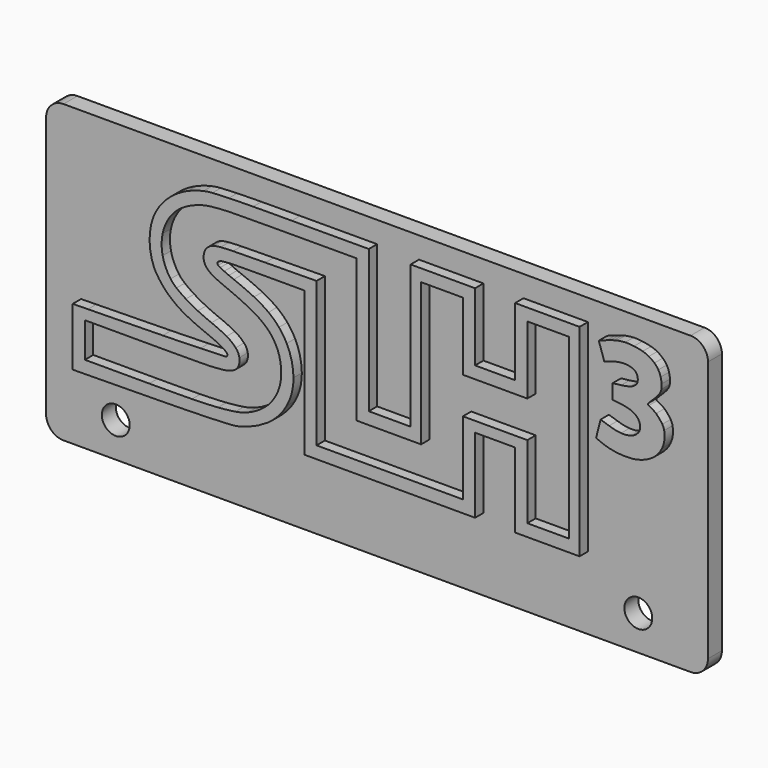
from build123d import *

# Parameters (mm, degrees)
F1_DEPTH = 6
F2_W     = 380
F2_H     = 170
F2_R     = 8
F3_DEPTH = 10
F4_R     = 10


# Not quite as in the source:
# - ends of sketch curves that miss each other by under 0.0002 mm in the source are joined


with BuildPart() as f1:
    # F0 (on Front) → F1 (new body)
    with BuildSketch(Plane.XZ):
        with BuildLine():
            ThreePointArc((152.341228018, 58.1349171313), (149.8269064082, 58.3597525344), (147.3038345575, 58.4402047098))
            ThreePointArc((147.3038345575, 58.4402047098), (144.8923426463, 58.2191881424), (142.5041551762, 57.818311393))
            ThreePointArc((142.5041551762, 57.818311393), (141.6286371814, 57.5874283564), (140.7541334629, 57.352732867))
            ThreePointArc((140.7541334629, 57.352732867), (139.7941303297, 57.0530705945), (138.8354301453, 56.749265641))
            ThreePointArc((138.8354301453, 56.749265641), (137.8311964898, 56.4206441356), (136.8284840268, 56.0874099159))
            ThreePointArc((136.8284840268, 56.0874099159), (134.4494339346, 55.2578316154), (132.1058124304, 54.3328896165))
            Line((132.1058124304, 54.3328896165), (135.2964043617, 44.7889044881))
            ThreePointArc((135.2964043617, 44.7889044881), (138.9218950311, 46.1431942866), (142.6777168508, 47.0770496879))
            ThreePointArc((142.6777168508, 47.0770496879), (145.3037154455, 47.4599296937), (147.9574100047, 47.4791820766))
            ThreePointArc((147.9574100047, 47.4791820766), (150.0024260919, 47.1622128392), (151.9545679078, 46.4754067993))
            ThreePointArc((151.9545679078, 46.4754067993), (153.2497169486, 45.5413952884), (154.0946016381, 44.1864198624))
            ThreePointArc((154.0946016381, 44.1864198624), (154.4618796803, 42.6793722604), (154.4471411344, 41.1282859819))
            ThreePointArc((154.4471411344, 41.1282859819), (154.0274505966, 39.8196352665), (153.1810760747, 38.7368809167))
            ThreePointArc((153.1810760747, 38.7368809167), (151.7322273647, 37.7109786626), (150.0881481192, 37.0411715732))
            ThreePointArc((150.0881481192, 37.0411715732), (147.5640252841, 36.4404230958), (145.0010969923, 36.0360800651))
            Line((145.0010969923, 36.0360800651), (140.077451, 35.452947))
            Line((140.077451, 35.452947), (140.077451, 31.231529))
            Line((140.077451, 31.231529), (140.077451, 27.010111))
            Line((140.077451, 27.010111), (145.313272, 26.390005))
            ThreePointArc((145.313272, 26.390005), (147.4995114305, 26.0344391507), (149.6467600868, 25.4909382897))
            ThreePointArc((149.6467600868, 25.4909382897), (151.3253195044, 24.8379266625), (152.8788301944, 23.9265592779))
            ThreePointArc((152.8788301944, 23.9265592779), (154.0260482227, 22.9373393661), (154.9508350367, 21.7375750228))
            ThreePointArc((154.9508350367, 21.7375750228), (155.5731072533, 20.4211762125), (155.8821842516, 18.9982919249))
            ThreePointArc((155.8821842516, 18.9982919249), (155.6792998869, 16.9086609443), (154.6903602154, 15.0567108232))
            ThreePointArc((154.6903602154, 15.0567108232), (152.9583603485, 13.4737955374), (150.8501020813, 12.4438967473))
            ThreePointArc((150.8501020813, 12.4438967473), (147.9002641766, 11.809008744), (144.8831400017, 11.7691580196))
            ThreePointArc((144.8831400017, 11.7691580196), (141.4066010267, 12.2925822347), (138.0238769802, 13.2504309438))
            Line((138.0238769802, 13.2504309438), (133.1239811244, 14.812147956))
            Line((133.1239811244, 14.812147956), (130.5830776691, 4.6951826662))
            ThreePointArc((130.5830776691, 4.6951826662), (134.3545111151, 3.0830213335), (138.2702710743, 1.8625303084))
            ThreePointArc((138.2702710743, 1.8625303084), (144.6475148349, 0.8652287383), (151.1020819971, 0.9143360329))
            ThreePointArc((151.1020819971, 0.9143360329), (156.7168065495, 2.0783580357), (161.91616203, 4.4963699511))
            ThreePointArc((161.91616203, 4.4963699511), (165.7064525048, 7.6555621469), (168.4426272472, 11.7616728825))
            ThreePointArc((168.4426272472, 11.7616728825), (169.7953031287, 16.3544948874), (169.6605109651, 21.1404719934))
            ThreePointArc((169.6605109651, 21.1404719934), (169.2435398041, 22.6044121534), (168.5656666596, 23.9673037896))
            ThreePointArc((168.5656666596, 23.9673037896), (166.9064128382, 26.1972938101), (165.0162637234, 28.2352622598))
            ThreePointArc((165.0162637234, 28.2352622598), (162.9669138924, 29.6544963373), (160.7904410002, 30.8698258589))
            ThreePointArc((160.7904410002, 30.8698258589), (160.3825279534, 31.451864804), (160.663634351, 32.1046600097))
            ThreePointArc((160.663634351, 32.1046600097), (162.3630635173, 33.8079757087), (164.0774507347, 35.4962352653))
            ThreePointArc((164.0774507347, 35.4962352653), (165.1707236148, 36.6322034695), (166.2196933125, 37.809204732))
            ThreePointArc((166.2196933125, 37.809204732), (166.8414404287, 38.6357965203), (167.3527699769, 39.5348880112))
            ThreePointArc((167.3527699769, 39.5348880112), (167.8080801222, 40.4998853929), (168.087775057, 41.5295931274))
            ThreePointArc((168.087775057, 41.5295931274), (168.1977643706, 42.8800995541), (168.1963354349, 44.2350767553))
            ThreePointArc((168.1963354349, 44.2350767553), (167.9958020572, 45.8752345594), (167.6282000052, 47.4861970012))
            ThreePointArc((167.6282000052, 47.4861970012), (167.0891813187, 49.1526573167), (166.3039485131, 50.7182373082))
            ThreePointArc((166.3039485131, 50.7182373082), (165.2790917625, 52.1671747641), (164.0500026364, 53.4474447096))
            ThreePointArc((164.0500026364, 53.4474447096), (162.513830675, 54.6803953844), (160.8520869325, 55.7380338798))
            ThreePointArc((160.8520869325, 55.7380338798), (159.1271747087, 56.5645242409), (157.3094311562, 57.1596856085))
            ThreePointArc((157.3094311562, 57.1596856085), (154.8393231071, 57.7185897611), (152.341228018, 58.1349171313))
        make_face()
    extrude(amount=F1_DEPTH)


with BuildPart() as f1b:
    # F0 (on Front) → F1, piece 2 (new body)
    with BuildSketch(Plane.XZ):
        with BuildLine():
            ThreePointArc((-89.7158710092, 56.8834551585), (-92.2735942046, 56.6347400971), (-94.8042470377, 56.1879701736))
            ThreePointArc((-94.8042470377, 56.1879701736), (-99.3736938541, 54.9568862269), (-103.7987699924, 53.2793543903))
            ThreePointArc((-103.7987699924, 53.2793543903), (-107.8572904997, 51.2349120693), (-111.665558992, 48.7553104477))
            ThreePointArc((-111.665558992, 48.7553104477), (-115.0425226555, 45.9681171918), (-118.0767520571, 42.8112545453))
            ThreePointArc((-118.0767520571, 42.8112545453), (-121.12070834, 38.6532182392), (-123.4993151686, 34.0818764963))
            ThreePointArc((-123.4993151686, 34.0818764963), (-125.7717067995, 20.9710825795), (-123.0967220919, 7.9364695178))
            ThreePointArc((-123.0967220919, 7.9364695178), (-120.9885218169, 4.3857057485), (-118.5278910102, 1.0694235263))
            ThreePointArc((-118.5278910102, 1.0694235263), (-115.7462308189, -1.9692311529), (-112.6660909179, -4.7048835193))
            ThreePointArc((-112.6660909179, -4.7048835193), (-108.9951941367, -7.3754936141), (-105.0961528177, -9.7003846329))
            ThreePointArc((-105.0961528177, -9.7003846329), (-100.2941341921, -12.1054997132), (-95.3662908353, -14.2409905891))
            ThreePointArc((-95.3662908353, -14.2409905891), (-91.8421068748, -15.6870234447), (-88.3419598235, -17.1903045981))
            ThreePointArc((-88.3419598235, -17.1903045981), (-86.1529724976, -18.2297863885), (-84.0291443228, -19.3966375486))
            ThreePointArc((-84.0291443228, -19.3966375486), (-82.7599951917, -20.2264826141), (-81.5746631598, -21.172194182))
            ThreePointArc((-81.5746631598, -21.172194182), (-81.1710412365, -21.8195919106), (-81.1923597658, -22.5822060778))
            ThreePointArc((-81.1923597658, -22.5822060778), (-81.6047236673, -23.1553562233), (-82.2701210101, -23.3915577353))
            ThreePointArc((-82.2701210101, -23.3915577353), (-89.4196222871, -23.6529407729), (-96.5698990129, -23.8921735944))
            ThreePointArc((-96.5698990129, -23.8921735944), (-107.3762638319, -24.1981884626), (-118.1845449963, -24.426714213))
            ThreePointArc((-118.1845449963, -24.426714213), (-139.6783524604, -24.7922369482), (-161.1725489962, -25.1341162467))
            Line((-161.1725489962, -25.1341162467), (-169.922549, -25.268471))
            Line((-169.922549, -25.268471), (-169.922549, -41.902849))
            Line((-169.922549, -41.902849), (-169.922549, -58.537228))
            Line((-169.922549, -58.537228), (-125.172549, -58.013692))
            ThreePointArc((-125.172549, -58.013692), (-115.0424725161, -57.8782248746), (-104.9129060058, -57.7088636826))
            ThreePointArc((-104.9129060058, -57.7088636826), (-97.5129944762, -57.5418252197), (-90.114737023, -57.3129603439))
            ThreePointArc((-90.114737023, -57.3129603439), (-84.6913364364, -57.1009616803), (-79.2697880179, -56.8459516498))
            ThreePointArc((-79.2697880179, -56.8459516498), (-77.083403988, -56.6404610548), (-74.9225491136, -56.2490434966))
            ThreePointArc((-74.9225491136, -56.2490434966), (-66.2429199717, -53.4275060959), (-58.229199749, -49.0597463737))
            ThreePointArc((-58.229199749, -49.0597463737), (-51.8949561555, -43.6034600395), (-47.0349944418, -36.8009257582))
            ThreePointArc((-47.0349944418, -36.8009257582), (-44.1187465301, -29.3501508182), (-43.1776257233, -21.4045329973))
            ThreePointArc((-43.1776257233, -21.4045329973), (-44.2002643647, -13.1406454463), (-47.0554066795, -5.3185108399))
            ThreePointArc((-47.0554066795, -5.3185108399), (-49.0771830946, -1.8182961093), (-51.5059305748, 1.4128443618))
            ThreePointArc((-51.5059305748, 1.4128443618), (-54.3478662536, 4.3900005354), (-57.5111356244, 7.0232085076))
            ThreePointArc((-57.5111356244, 7.0232085076), (-61.5514455995, 9.7367639846), (-65.8219646825, 12.0713206495))
            ThreePointArc((-65.8219646825, 12.0713206495), (-71.5688253864, 14.7325295165), (-77.4225488118, 17.1496274843))
            ThreePointArc((-77.4225488118, 17.1496274843), (-78.8401462889, 17.7131254267), (-80.2487799398, 18.2986711417))
            ThreePointArc((-80.2487799398, 18.2986711417), (-81.6057167765, 18.888922599), (-82.9523677552, 19.5022785255))
            ThreePointArc((-82.9523677552, 19.5022785255), (-84.0942604495, 20.0454792956), (-85.2272229395, 20.6070681197))
            ThreePointArc((-85.2272229395, 20.6070681197), (-85.8377507575, 20.9485781165), (-86.4176780147, 21.3398039801))
            ThreePointArc((-86.4176780147, 21.3398039801), (-86.853730235, 22.0915551847), (-86.6016505259, 22.9232565972))
            ThreePointArc((-86.6016505259, 22.9232565972), (-85.6588933579, 23.6905603449), (-84.5036700444, 24.0687213317))
            ThreePointArc((-84.5036700444, 24.0687213317), (-80.9344247322, 24.4386370453), (-77.3495189905, 24.5961183335))
            ThreePointArc((-77.3495189905, 24.5961183335), (-69.2612379194, 24.6836352737), (-61.1725489995, 24.7162152783))
            Line((-61.1725489995, 24.7162152783), (-36.922549, 24.731529))
            Line((-36.922549, 24.731529), (-36.922549, -16.768471))
            Line((-36.922549, -16.768471), (-36.922549, -58.268471))
            Line((-36.922549, -58.268471), (12.077451, -58.268471))
            Line((12.077451, -58.268471), (61.077451, -58.268471))
            Line((61.077451, -58.268471), (61.077451, -36.768471))
            Line((61.077451, -36.768471), (61.077451, -15.268471))
            Line((61.077451, -15.268471), (72.577451, -15.268471))
            Line((72.577451, -15.268471), (84.077451, -15.268471))
            Line((84.077451, -15.268471), (84.077451, -36.768471))
            Line((84.077451, -36.768471), (84.077451, -58.268471))
            Line((84.077451, -58.268471), (102.577451, -58.268471))
            Line((102.577451, -58.268471), (121.077451, -58.268471))
            Line((121.077451, -58.268471), (121.077451, -0.268471))
            Line((121.077451, -0.268471), (121.077451, 57.731529))
            Line((121.077451, 57.731529), (102.577451, 57.731529))
            Line((102.577451, 57.731529), (84.077451, 57.731529))
            Line((84.077451, 57.731529), (84.077451, 38.231529))
            Line((84.077451, 38.231529), (84.077451, 18.731529))
            Line((84.077451, 18.731529), (72.577451, 18.731529))
            Line((72.577451, 18.731529), (61.077451, 18.731529))
            Line((61.077451, 18.731529), (61.077451, 38.231529))
            Line((61.077451, 38.231529), (61.077451, 57.731529))
            Line((61.077451, 57.731529), (42.577451, 57.731529))
            Line((42.577451, 57.731529), (24.077451, 57.731529))
            Line((24.077451, 57.731529), (24.077451, 16.731529))
            Line((24.077451, 16.731529), (24.077451, -24.268471))
            Line((24.077451, -24.268471), (12.077451, -24.268471))
            Line((12.077451, -24.268471), (0.077451, -24.268471))
            Line((0.077451, -24.268471), (0.077451, 16.731529))
            Line((0.077451, 16.731529), (0.077451, 57.731529))
            Line((0.077451, 57.731529), (-44.172549, 57.652029))
            ThreePointArc((-44.172549, 57.652029), (-55.2418806461, 57.6161162906), (-66.3110620044, 57.5481685759))
            ThreePointArc((-66.3110620044, 57.5481685759), (-73.3088995976, 57.4577720999), (-80.3053760072, 57.2927862479))
            ThreePointArc((-80.3053760072, 57.2927862479), (-85.0121136593, 57.1223791714), (-89.7158710092, 56.8834551585))
        make_face()
        with BuildLine():
            Line((-6.922549, 50.731529), (-6.922549, 9.731529))
            Line((-6.922549, 9.731529), (-6.922549, -31.268471))
            Line((-6.922549, -31.268471), (11.577451, -31.268471))
            Line((11.577451, -31.268471), (30.077451, -31.268471))
            Line((30.077451, -31.268471), (30.077451, 9.731529))
            Line((30.077451, 9.731529), (30.077451, 50.731529))
            Line((30.077451, 50.731529), (42.077451, 50.731529))
            Line((42.077451, 50.731529), (54.077451, 50.731529))
            Line((54.077451, 50.731529), (54.077451, 31.231529))
            Line((54.077451, 31.231529), (54.077451, 11.731529))
            Line((54.077451, 11.731529), (72.577451, 11.731529))
            Line((72.577451, 11.731529), (91.077451, 11.731529))
            Line((91.077451, 11.731529), (91.077451, 31.231529))
            Line((91.077451, 31.231529), (91.077451, 50.731529))
            Line((91.077451, 50.731529), (103.077451, 50.731529))
            Line((103.077451, 50.731529), (115.077451, 50.731529))
            Line((115.077451, 50.731529), (115.077451, -0.268471))
            Line((115.077451, -0.268471), (115.077451, -51.268471))
            Line((115.077451, -51.268471), (103.077451, -51.268471))
            Line((103.077451, -51.268471), (91.077451, -51.268471))
            Line((91.077451, -51.268471), (91.077451, -30.268471))
            Line((91.077451, -30.268471), (91.077451, -9.268471))
            Line((91.077451, -9.268471), (72.577451, -9.268471))
            Line((72.577451, -9.268471), (54.077451, -9.268471))
            Line((54.077451, -9.268471), (54.077451, -30.268471))
            Line((54.077451, -30.268471), (54.077451, -51.268471))
            Line((54.077451, -51.268471), (12.077451, -51.268471))
            Line((12.077451, -51.268471), (-29.922549, -51.268471))
            Line((-29.922549, -51.268471), (-29.922549, -9.712924))
            Line((-29.922549, -9.712924), (-29.922549, 31.842624))
            Line((-29.922549, 31.842624), (-59.351393, 31.537076))
            ThreePointArc((-59.351393, 31.537076), (-68.5850462649, 31.4296314933), (-77.8184010104, 31.2990286783))
            ThreePointArc((-77.8184010104, 31.2990286783), (-81.409671871, 31.1906978742), (-84.9961810646, 30.9764228658))
            ThreePointArc((-84.9961810646, 30.9764228658), (-86.9969034513, 30.7468714781), (-88.9730370675, 30.3589542835))
            ThreePointArc((-88.9730370675, 30.3589542835), (-90.3497041231, 29.8794538341), (-91.6013931015, 29.1321871364))
            ThreePointArc((-91.6013931015, 29.1321871364), (-92.2881410377, 28.5718283118), (-92.9221711737, 27.9524491626))
            ThreePointArc((-92.9221711737, 27.9524491626), (-93.4234380719, 27.3440152924), (-93.8438617689, 26.677153874))
            ThreePointArc((-93.8438617689, 26.677153874), (-94.1817162815, 25.9538613819), (-94.4271884372, 25.1942291118))
            ThreePointArc((-94.4271884372, 25.1942291118), (-94.6171600755, 24.2984091052), (-94.7324511912, 23.3899540163))
            ThreePointArc((-94.7324511912, 23.3899540163), (-94.6898825108, 21.7428303685), (-94.2866406888, 20.1452621164))
            ThreePointArc((-94.2866406888, 20.1452621164), (-93.5430426827, 18.6793780125), (-92.4936754461, 17.414236537))
            ThreePointArc((-92.4936754461, 17.414236537), (-90.8288592178, 16.0278457455), (-88.9812839954, 14.8964050088))
            ThreePointArc((-88.9812839954, 14.8964050088), (-86.0853857569, 13.4838421599), (-83.127087951, 12.2071141212))
            ThreePointArc((-83.127087951, 12.2071141212), (-76.1046774408, 9.2216982414), (-69.192652154, 5.9889186855))
            ThreePointArc((-69.192652154, 5.9889186855), (-64.6346128235, 3.4496167949), (-60.3711449209, 0.4418571004))
            ThreePointArc((-60.3711449209, 0.4418571004), (-57.3596650438, -2.3287384368), (-54.8044534441, -5.5250026212))
            ThreePointArc((-54.8044534441, -5.5250026212), (-52.7953245926, -9.0398392377), (-51.3626788706, -12.8264209624))
            ThreePointArc((-51.3626788706, -12.8264209624), (-50.3291791157, -18.119537933), (-50.2608906295, -23.5121759512))
            ThreePointArc((-50.2608906295, -23.5121759512), (-51.1807718794, -28.6284665045), (-53.1033518636, -33.4581970709))
            ThreePointArc((-53.1033518636, -33.4581970709), (-55.9945311141, -37.8976652666), (-59.6944190526, -41.6895809375))
            ThreePointArc((-59.6944190526, -41.6895809375), (-64.2892009878, -44.9586351909), (-69.3529080105, -47.4400879732))
            ThreePointArc((-69.3529080105, -47.4400879732), (-72.8684407738, -48.6039602475), (-76.4898430612, -49.3779206108))
            ThreePointArc((-76.4898430612, -49.3779206108), (-81.4935417039, -50.0516975389), (-86.5221440209, -50.5035096908))
            ThreePointArc((-86.5221440209, -50.5035096908), (-93.9698805478, -50.9055572117), (-101.4257790076, -51.1055564262))
            ThreePointArc((-101.4257790076, -51.1055564262), (-113.71007347, -51.2277373319), (-125.994908, -51.2684709995))
            Line((-125.994908, -51.2684709995), (-162.922549, -51.268471))
            Line((-162.922549, -51.268471), (-162.922549, -41.268471))
            Line((-162.922549, -41.268471), (-162.922549, -31.268471))
            Line((-162.922549, -31.268471), (-122.89043, -31.268471))
            ThreePointArc((-122.89043, -31.268471), (-108.6116969212, -31.2385282409), (-94.333215, -31.148701002))
            ThreePointArc((-94.333215, -31.148701002), (-88.8830809379, -30.9627118289), (-83.4497240276, -30.4966797533))
            ThreePointArc((-83.4497240276, -30.4966797533), (-80.5892836984, -29.9451631776), (-77.8516171162, -28.9494367453))
            ThreePointArc((-77.8516171162, -28.9494367453), (-76.0486360653, -27.6977755498), (-74.7978693807, -25.8941738265))
            ThreePointArc((-74.7978693807, -25.8941738265), (-74.163782837, -23.6465963892), (-74.2341387938, -21.3123469619))
            ThreePointArc((-74.2341387938, -21.3123469619), (-74.9963742674, -19.0247201541), (-76.3569290939, -17.0339590855))
            ThreePointArc((-76.3569290939, -17.0339590855), (-78.7940710577, -14.772962488), (-81.5764459433, -12.9535788949))
            ThreePointArc((-81.5764459433, -12.9535788949), (-85.8570506833, -10.8047203157), (-90.2567551169, -8.9116352955))
            ThreePointArc((-90.2567551169, -8.9116352955), (-94.2221619869, -7.2543553332), (-98.1217563571, -5.4476477338))
            ThreePointArc((-98.1217563571, -5.4476477338), (-101.5861180366, -3.6519049869), (-104.9550017172, -1.6828655431))
            ThreePointArc((-104.9550017172, -1.6828655431), (-107.7122197443, 0.1346344078), (-110.3613500245, 2.106350969))
            ThreePointArc((-110.3613500245, 2.106350969), (-112.1670046714, 3.7461922987), (-113.7300718859, 5.6187010826))
            ThreePointArc((-113.7300718859, 5.6187010826), (-116.5390282465, 10.4950047459), (-118.280515566, 15.8462470928))
            ThreePointArc((-118.280515566, 15.8462470928), (-118.8790101532, 21.4407000717), (-118.3086948317, 27.0380959649))
            ThreePointArc((-118.3086948317, 27.0380959649), (-116.5989502708, 32.3696733886), (-113.8179953448, 37.2292242485))
            ThreePointArc((-113.8179953448, 37.2292242485), (-110.1022751062, 41.3715968897), (-105.5938670631, 44.6335111102))
            ThreePointArc((-105.5938670631, 44.6335111102), (-101.8608058475, 46.5327187651), (-97.9596561103, 48.0571093289))
            ThreePointArc((-97.9596561103, 48.0571093289), (-94.0658785153, 49.1295336068), (-90.0782940356, 49.7704453392))
            ThreePointArc((-90.0782940356, 49.7704453392), (-83.9399176718, 50.2700740279), (-77.7848659949, 50.4813365343))
            ThreePointArc((-77.7848659949, 50.4813365343), (-62.9789210123, 50.6078184187), (-48.1725489998, 50.6657178536))
            Line((-48.1725489998, 50.6657178536), (-6.922549, 50.731529))
        make_face(mode=Mode.SUBTRACT)
    extrude(amount=F1_DEPTH)


with BuildPart() as f3:
    # F2 (on Front) → F3 (new body)
    with BuildSketch(Plane.XZ):
        with Locations((0, -15)):
            Rectangle(F2_W, F2_H)
        with Locations((-150, -80)):
            Circle(F2_R, mode=Mode.SUBTRACT)
        with Locations((150, -80)):
            Circle(F2_R, mode=Mode.SUBTRACT)
    extrude(amount=-F3_DEPTH)

    # F4
    f4_edges = [f3.edges().sort_by_distance(p)[0] for p in [
        (-190, 5, 70),
        (-190, 5, -100),
        (190, 5, -100),
        (190, 5, 70),
    ]]
    fillet(f4_edges, radius=F4_R)


solid = Compound([f1.part, f1b.part, f3.part])
